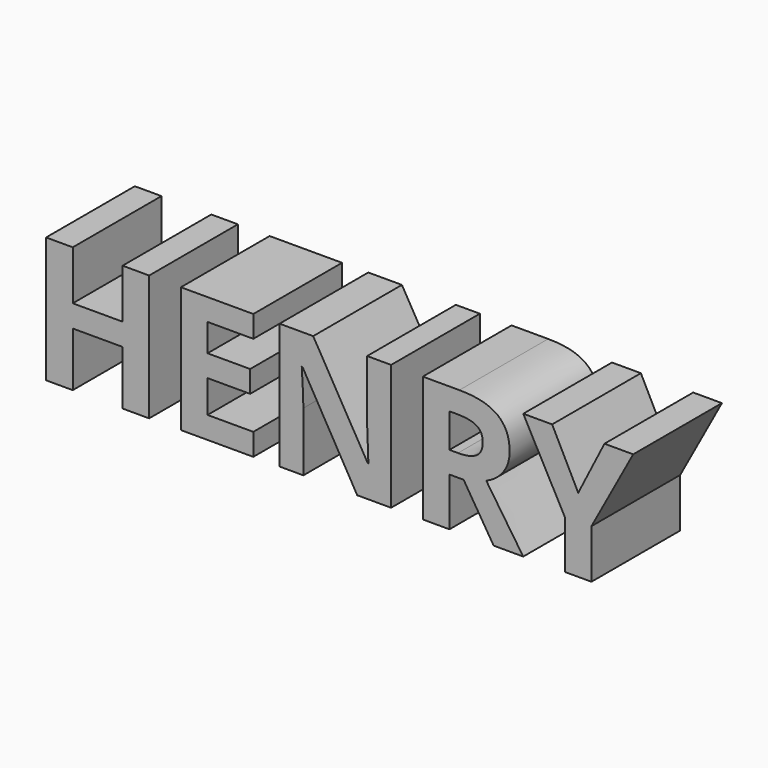
from build123d import *

# Parameters (mm, degrees)
F0_TEXT_SIZE = 39.7108417625
F1_DEPTH     = 25


# Not quite as in the source:
# - Text() gives the source's letters only with a copy of the font that has no kerning and outlines rounded to 1/6400 em; it was checked with that copy


with BuildPart() as f1:
    # F0 (on Front) → F1 (new body)
    with BuildSketch(Plane.XZ):
        with Locations((-61.7583021522, 0)):
            Text('HENRY', F0_TEXT_SIZE, font='Open Sans', font_style=FontStyle.BOLD, text_align=(TextAlign.LEFT, TextAlign.BOTTOM))
    extrude(amount=F1_DEPTH)


solid = f1.part
